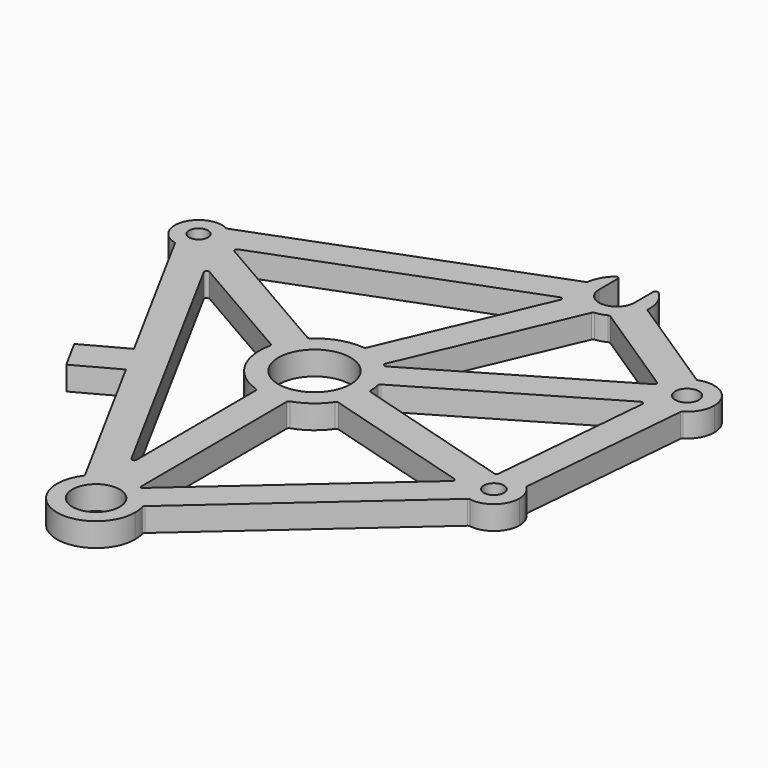
from build123d import *

# Parameters (mm, degrees)
F1_R        = 0.8
F1_R_2      = 1.5
F1_R_3      = 1
F1_R_4      = 0.85
F1_R_5      = 2
F1_R_6      = 3.05
F2_DEPTH    = 2
F4_DEPTH    = 2.001
F5_T1_DEPTH = 2
F5_T3_DEPTH = 4.0603808135


# Not quite as in the source:
# - a fillet or chamfer that OpenCascade refuses, or shapes differently, is made with other operations: its cross-section is extruded or revolved along the edge and cut away or added


with BuildPart() as f2:
    # F1 (on Top) → F2 (new body)
    with BuildSketch(Plane.XY):
        with BuildLine():
            ThreePointArc((5.1588517672, 41.7551647468), (5.8189357702, 41.1743283067), (6.1661273036, 40.3665288884))
            Line((6.1661273036, 40.3665288884), (7.2214972283, 39.7576616241))
            Line((7.2214972283, 39.7576616241), (28.9007343827, 47.9973716865))
            Line((28.9007343827, 47.9973716865), (29.1292494513, 48.531429375))
            ThreePointArc((29.1292494513, 48.531429375), (28.6106135221, 49.5207693713), (28.5200074656, 50.6341279828))
            Line((28.5200074656, 50.6341279828), (5.1588517672, 41.7551647468))
        make_face()
        with BuildLine():
            Line((42.9265921342, 44.2277120811), (34.0866325696, 50.0267255555))
            ThreePointArc((34.0866325696, 50.0267255555), (33.6412025938, 48.7641710985), (32.6605057325, 47.8527517184))
            Line((32.6605057325, 47.8527517184), (41.3390492003, 42.1596272035))
            Line((41.3390492003, 42.1596272035), (41.5054041139, 42.257574489))
            ThreePointArc((41.5054041139, 42.257574489), (41.9346789885, 43.4455770228), (42.9265921342, 44.2277120811))
        make_face()
        with BuildLine():
            Line((43.6434620305, 25.2933980565), (44.9307446243, 40.097147885))
            ThreePointArc((44.9307446243, 40.097147885), (43.8873688977, 39.8016600174), (42.8245714122, 40.0170839983))
            Line((42.8245714122, 40.0170839983), (42.2864184602, 39.7002275873))
            Line((42.2864184602, 39.7002275873), (41.0532365012, 25.518635059))
            ThreePointArc((41.0532365012, 25.518635059), (42.3862536752, 25.8419172646), (43.6434620305, 25.2933980565))
        make_face()
        with BuildLine():
            Line((39.5736067493, 23.1147203388), (23.9127614663, 9.2822986167))
            ThreePointArc((23.9127614663, 9.2822986167), (24.9733654225, 8.4845968706), (25.6339590007, 7.3335864657))
            Line((25.6339590007, 7.3335864657), (41.7771062071, 21.5920007495))
            ThreePointArc((41.7771062071, 21.5920007495), (40.8113081392, 22.0586484485), (40.1911511893, 22.9338234826))
            Line((40.1911511893, 22.9338234826), (39.5736067493, 23.1147203388))
        make_face()
        with BuildLine():
            ThreePointArc((6.0825746745, 39.3247870004), (6.1704249985, 39.6573262113), (6.2, 40))
            ThreePointArc((6.2, 40), (6.1915138221, 40.184045365), (6.1661273036, 40.3665288884))
            ThreePointArc((6.1661273036, 40.3665288884), (5.8189357702, 41.1743283067), (5.1588517672, 41.7551647468))
            ThreePointArc((5.1588517672, 41.7551647468), (2.3247456616, 40.6952849534), (3.782863546, 38.0439843613))
            ThreePointArc((3.782863546, 38.0439843613), (4.3297316575, 38.004212011), (4.8668489245, 38.1144463646))
            ThreePointArc((4.8668489245, 38.1144463646), (5.5958497172, 38.5676580133), (6.0677200026, 39.2847224372))
            ThreePointArc((6.0677200026, 39.2847224372), (6.0752543384, 39.3047150466), (6.0825746745, 39.3247870004))
        make_face()
        with Locations((4.2, 40)):
            Circle(F1_R, mode=Mode.SUBTRACT)
        with BuildLine():
            ThreePointArc((34.1, 50.3), (31.4673632334, 53.094993658), (28.5200074656, 50.6341279828))
            ThreePointArc((28.5200074656, 50.6341279828), (28.6106135221, 49.5207693713), (29.1292494513, 48.531429375))
            ThreePointArc((29.1292494513, 48.531429375), (29.2798350863, 48.3612030221), (29.443730373, 48.2037502363))
            ThreePointArc((29.443730373, 48.2037502363), (30.4109250017, 47.6449019515), (31.5196205494, 47.5086263571))
            ThreePointArc((31.5196205494, 47.5086263571), (32.1085822981, 47.6192921332), (32.6605057325, 47.8527517184))
            ThreePointArc((32.6605057325, 47.8527517184), (33.6412025938, 48.7641710985), (34.0866325696, 50.0267255555))
            ThreePointArc((34.0866325696, 50.0267255555), (34.0966561457, 50.1631994059), (34.1, 50.3))
        make_face()
        with Locations((31.3, 50.3)):
            Circle(F1_R_2, mode=Mode.SUBTRACT)
        with BuildLine():
            ThreePointArc((46.1, 42.1), (45.080851652, 44.0103452687), (42.9265921342, 44.2277120811))
            ThreePointArc((42.9265921342, 44.2277120811), (41.9346789885, 43.4455770228), (41.5054041139, 42.257574489))
            ThreePointArc((41.5054041139, 42.257574489), (41.5006748227, 42.155711122), (41.5004652971, 42.053738244))
            ThreePointArc((41.5004652971, 42.053738244), (41.730713723, 41.0959809246), (42.340519095, 40.3223848876))
            ThreePointArc((42.340519095, 40.3223848876), (42.5730125438, 40.1546204015), (42.8245714122, 40.0170839983))
            ThreePointArc((42.8245714122, 40.0170839983), (43.8873688977, 39.8016600174), (44.9307446243, 40.097147885))
            ThreePointArc((44.9307446243, 40.097147885), (45.7862921029, 40.9404122793), (46.1, 42.1))
        make_face()
        with Locations((43.8, 42.1)):
            Circle(F1_R_3, mode=Mode.SUBTRACT)
        with BuildLine():
            ThreePointArc((40.1911511893, 22.9338234826), (40.8113081392, 22.0586484485), (41.7771062071, 21.5920007495))
            ThreePointArc((41.7771062071, 21.5920007495), (43.5625854735, 22.0369122611), (44.35, 23.7))
            ThreePointArc((44.35, 23.7), (44.1654443983, 24.5715092181), (43.6434620305, 25.2933980565))
            ThreePointArc((43.6434620305, 25.2933980565), (42.3862536752, 25.8419172646), (41.0532365012, 25.518635059))
            ThreePointArc((41.0532365012, 25.518635059), (40.9868167512, 25.475017297), (40.9220541458, 25.4289749546))
            ThreePointArc((40.9220541458, 25.4289749546), (40.2457819942, 24.5963994566), (40.0559086727, 23.5407129006))
            ThreePointArc((40.0559086727, 23.5407129006), (40.1014751279, 23.2323533801), (40.1911511893, 22.9338234826))
        make_face()
        with Locations((42.2, 23.7)):
            Circle(F1_R_4, mode=Mode.SUBTRACT)
        with BuildLine():
            ThreePointArc((22.1949878763, 9.5858739483), (21.6807151801, 9.4966814642), (21.1869382745, 9.3275186052))
            ThreePointArc((21.1869382745, 9.3275186052), (20.4876667271, 8.9154377834), (19.9101314198, 8.3451358725))
            ThreePointArc((19.9101314198, 8.3451358725), (21.4175412975, 3.1825838973), (25.8, 6.3))
            ThreePointArc((25.8, 6.3), (25.7582253377, 6.8234191904), (25.6339590007, 7.3335864657))
            ThreePointArc((25.6339590007, 7.3335864657), (24.9733654225, 8.4845968706), (23.9127614663, 9.2822986167))
            ThreePointArc((23.9127614663, 9.2822986167), (23.8501326105, 9.3111695293), (23.786914122, 9.3387253977))
            ThreePointArc((23.786914122, 9.3387253977), (23.0062642444, 9.5609349142), (22.1949878763, 9.5858739483))
        make_face()
        with Locations((22.5, 6.3)):
            Circle(F1_R_5, mode=Mode.SUBTRACT)
        with BuildLine():
            Line((7.2214972283, 39.7576616241), (6.0825746745, 39.3247870004))
            ThreePointArc((6.0825746745, 39.3247870004), (6.0752543384, 39.3047150466), (6.0677200026, 39.2847224372))
            Line((6.0677200026, 39.2847224372), (7.5409732288, 36.5716823429))
            Line((7.5409732288, 36.5716823429), (17.8832035005, 30.6050110324))
            ThreePointArc((17.8832035005, 30.6050110324), (18.3722370249, 31.8237094087), (19.1824818795, 32.8570935561))
            Line((19.1824818795, 32.8570935561), (7.2214972283, 39.7576616241))
        make_face()
        with BuildLine():
            ThreePointArc((6.1661273036, 40.3665288884), (6.1915138221, 40.184045365), (6.2, 40))
            ThreePointArc((6.2, 40), (6.1704249985, 39.6573262113), (6.0825746745, 39.3247870004))
            Line((6.0825746745, 39.3247870004), (7.2214972283, 39.7576616241))
            Line((7.2214972283, 39.7576616241), (6.1661273036, 40.3665288884))
        make_face()
        with BuildLine():
            Line((7.5409732288, 36.5716823429), (6.0677200026, 39.2847224372))
            ThreePointArc((6.0677200026, 39.2847224372), (5.5958497172, 38.5676580133), (4.8668489245, 38.1144463646))
            Line((4.8668489245, 38.1144463646), (7.5409732288, 36.5716823429))
        make_face()
        with BuildLine():
            ThreePointArc((4.8668489245, 38.1144463646), (4.3297316575, 38.004212011), (3.782863546, 38.0439843613))
            Line((3.782863546, 38.0439843613), (11.1306870545, 24.5127465342))
            Line((11.1306870545, 24.5127465342), (12.5623079112, 21.8763736997))
            Line((12.5623079112, 21.8763736997), (19.9101314198, 8.3451358725))
            ThreePointArc((19.9101314198, 8.3451358725), (20.4876667271, 8.9154377834), (21.1869382745, 9.3275186052))
            Line((21.1869382745, 9.3275186052), (21.1777502182, 11.4591476685))
            Line((21.1777502182, 11.4591476685), (7.5409732288, 36.5716823429))
            Line((7.5409732288, 36.5716823429), (4.8668489245, 38.1144463646))
        make_face()
        with BuildLine():
            Line((22.1949878763, 9.5858739483), (21.1777502182, 11.4591476685))
            Line((21.1777502182, 11.4591476685), (21.1869382745, 9.3275186052))
            ThreePointArc((21.1869382745, 9.3275186052), (21.6807151801, 9.4966814642), (22.1949878763, 9.5858739483))
        make_face()
        with BuildLine():
            Line((21.119255789, 25.0298552298), (21.1777502182, 11.4591476685))
            Line((21.1777502182, 11.4591476685), (22.1949878763, 9.5858739483))
            ThreePointArc((22.1949878763, 9.5858739483), (23.0062642444, 9.5609349142), (23.786914122, 9.3387253977))
            Line((23.786914122, 9.3387253977), (23.7192316366, 25.0410620223))
            ThreePointArc((23.7192316366, 25.0410620223), (22.4200429173, 24.8500431957), (21.119255789, 25.0298552298))
        make_face()
        with BuildLine():
            Line((40.0559086727, 23.5407129006), (39.5736067493, 23.1147203388))
            Line((39.5736067493, 23.1147203388), (40.1911511893, 22.9338234826))
            ThreePointArc((40.1911511893, 22.9338234826), (40.1014751279, 23.2323533801), (40.0559086727, 23.5407129006))
        make_face()
        with BuildLine():
            ThreePointArc((27.0499939641, 29.4925077351), (26.8624824403, 28.192808174), (26.3190910076, 26.9973562631))
            Line((26.3190910076, 26.9973562631), (39.5736067493, 23.1147203388))
            Line((39.5736067493, 23.1147203388), (40.0559086727, 23.5407129006))
            ThreePointArc((40.0559086727, 23.5407129006), (40.2457819942, 24.5963994566), (40.9220541458, 25.4289749546))
            Line((40.9220541458, 25.4289749546), (27.0499939641, 29.4925077351))
        make_face()
        with BuildLine():
            Line((29.1292494513, 48.531429375), (28.9007343827, 47.9973716865))
            Line((28.9007343827, 47.9973716865), (29.443730373, 48.2037502363))
            ThreePointArc((29.443730373, 48.2037502363), (29.2798350863, 48.3612030221), (29.1292494513, 48.531429375))
        make_face()
        with BuildLine():
            Line((29.443730373, 48.2037502363), (28.9007343827, 47.9973716865))
            Line((28.9007343827, 47.9973716865), (22.9611178394, 34.116020664))
            ThreePointArc((22.9611178394, 34.116020664), (24.229243859, 33.7750867716), (25.3514889375, 33.0932176461))
            Line((25.3514889375, 33.0932176461), (31.5196205494, 47.5086263571))
            ThreePointArc((31.5196205494, 47.5086263571), (30.4109250017, 47.6449019515), (29.443730373, 48.2037502363))
        make_face()
        with BuildLine():
            ThreePointArc((22.9611178394, 34.116020664), (20.9301904957, 33.9115938187), (19.1824818795, 32.8570935561))
            ThreePointArc((19.1824818795, 32.8570935561), (18.3722370249, 31.8237094087), (17.8832035005, 30.6050110324))
            ThreePointArc((17.8832035005, 30.6050110324), (18.378375934, 27.1656821399), (21.119255789, 25.0298552298))
            ThreePointArc((21.119255789, 25.0298552298), (22.4200429173, 24.8500431957), (23.7192316366, 25.0410620223))
            ThreePointArc((23.7192316366, 25.0410620223), (25.1958501069, 25.7843947761), (26.3190910076, 26.9973562631))
            ThreePointArc((26.3190910076, 26.9973562631), (26.8624824403, 28.192808174), (27.0499939641, 29.4925077351))
            ThreePointArc((27.0499939641, 29.4925077351), (27.049998491, 29.4962538663), (27.05, 29.5))
            ThreePointArc((27.05, 29.5), (27.0140701204, 30.0769375391), (26.9068357316, 30.6449592518))
            ThreePointArc((26.9068357316, 30.6449592518), (26.40703107, 31.8592799758), (25.5876684333, 32.8854497425))
            ThreePointArc((25.5876684333, 32.8854497425), (25.471336058, 32.991331382), (25.3514889375, 33.0932176461))
            ThreePointArc((25.3514889375, 33.0932176461), (24.229243859, 33.7750867716), (22.9611178394, 34.116020664))
        make_face()
        with Locations((22.4, 29.5)):
            Circle(F1_R_6, mode=Mode.SUBTRACT)
        with BuildLine():
            Line((41.5054041139, 42.257574489), (41.3390492003, 42.1596272035))
            Line((41.3390492003, 42.1596272035), (41.5004652971, 42.053738244))
            ThreePointArc((41.5004652971, 42.053738244), (41.5006748227, 42.155711122), (41.5054041139, 42.257574489))
        make_face()
        with BuildLine():
            Line((42.340519095, 40.3223848876), (42.2864184602, 39.7002275873))
            Line((42.2864184602, 39.7002275873), (42.8245714122, 40.0170839983))
            ThreePointArc((42.8245714122, 40.0170839983), (42.5730125438, 40.1546204015), (42.340519095, 40.3223848876))
        make_face()
        with BuildLine():
            Line((41.3390492003, 42.1596272035), (25.5876684333, 32.8854497425))
            ThreePointArc((25.5876684333, 32.8854497425), (26.40703107, 31.8592799758), (26.9068357316, 30.6449592518))
            Line((26.9068357316, 30.6449592518), (42.2864184602, 39.7002275873))
            Line((42.2864184602, 39.7002275873), (42.340519095, 40.3223848876))
            ThreePointArc((42.340519095, 40.3223848876), (41.730713723, 41.0959809246), (41.5004652971, 42.053738244))
            Line((41.5004652971, 42.053738244), (41.3390492003, 42.1596272035))
        make_face()
        Polygon((12.5623079112, 21.8763736997), (11.1306870545, 24.5127465342), (7.6155232752, 22.6039187252), (9.0471441319, 19.9675458907), align=None)
    extrude(amount=-F2_DEPTH)

    # F3 (on face) → F4 (cut, through all)
    with BuildSketch(Plane.XY):
        with BuildLine():
            Line((29.8, 52.6643180835), (29.8, 50.3))
            ThreePointArc((29.8, 50.3), (31.3, 51.8), (32.8, 50.3))
            Line((32.8, 50.3), (32.8, 52.6643180835))
            ThreePointArc((32.8, 52.6643180835), (31.3, 53.1), (29.8, 52.6643180835))
        make_face()
    extrude(amount=-F4_DEPTH, mode=Mode.SUBTRACT)

    # F5: fillet of radius 0.2 on 35 edges, made by hand

    # F5_s2 → F5_t1 (join)
    with BuildSketch(Plane.XY.offset(-2)):
        with BuildLine():
            ThreePointArc((7.6152873474, 39.9073309314), (7.4869831486, 39.736368397), (7.586398465, 39.5471416799))
            Line((7.586398465, 39.5471416799), (7.2214972283, 39.7576616241))
            Line((7.2214972283, 39.7576616241), (7.6152873474, 39.9073309314))
        make_face()
        with BuildLine():
            ThreePointArc((8.1549136009, 36.2174859744), (7.9153841385, 36.1874830559), (7.8792109212, 35.9488074668))
            Line((7.8792109212, 35.9488074668), (7.5409732288, 36.5716823429))
            Line((7.5409732288, 36.5716823429), (8.1549136009, 36.2174859744))
        make_face()
        with BuildLine():
            ThreePointArc((20.7985689859, 12.157421304), (21.0239808003, 12.0591244239), (21.174325317, 12.2537247554))
            Line((21.174325317, 12.2537247554), (21.1777502182, 11.4591476685))
            Line((21.1777502182, 11.4591476685), (20.7985689859, 12.157421304))
        make_face()
        with BuildLine():
            ThreePointArc((19.8343096871, 8.2452750848), (19.8723110487, 8.349886538), (19.8485108874, 8.4586119349))
            Line((19.8485108874, 8.4586119349), (19.9101314198, 8.3451358725))
            ThreePointArc((19.9101314198, 8.3451358725), (19.8717462329, 8.295565618), (19.8343096871, 8.2452750848))
        make_face()
        with BuildLine():
            ThreePointArc((25.7307406523, 7.4190687367), (25.6711167797, 7.3250865393), (25.6709610076, 7.2137867848))
            ThreePointArc((25.6709610076, 7.2137867848), (25.6530290307, 7.273862378), (25.6339590007, 7.3335864657))
            Line((25.6339590007, 7.3335864657), (25.7307406523, 7.4190687367))
        make_face()
        with BuildLine():
            ThreePointArc((20.9809292738, 25.0718244983), (21.0812054105, 24.9995965527), (21.1198921159, 24.8822273979))
            Line((21.1198921159, 24.8822273979), (21.119255789, 25.0298552298))
            ThreePointArc((21.119255789, 25.0298552298), (21.0499294357, 25.0503023168), (20.9809292738, 25.0718244983))
        make_face()
        with BuildLine():
            ThreePointArc((17.7553292124, 30.6787846601), (17.8380565482, 30.5869785186), (17.85103896, 30.4640816648))
            ThreePointArc((17.85103896, 30.4640816648), (17.8665735681, 30.5346713424), (17.8832035005, 30.6050110324))
            Line((17.8832035005, 30.6050110324), (17.7553292124, 30.6787846601))
        make_face()
        with BuildLine():
            ThreePointArc((3.6998231735, 38.0635539919), (3.77290973, 38.0275334575), (3.8255636798, 37.9653507815))
            Line((3.8255636798, 37.9653507815), (3.782863546, 38.0439843613))
            ThreePointArc((3.782863546, 38.0439843613), (3.7412389988, 38.0533263387), (3.6998231735, 38.0635539919))
        make_face()
        with BuildLine():
            ThreePointArc((5.2424934778, 41.7869547697), (5.1620285352, 41.7741283656), (5.0831253359, 41.7944608218))
            ThreePointArc((5.0831253359, 41.7944608218), (5.1211981098, 41.7752166185), (5.1588517672, 41.7551647468))
            Line((5.1588517672, 41.7551647468), (5.2424934778, 41.7869547697))
        make_face()
        with BuildLine():
            ThreePointArc((28.4095590818, 50.5921494458), (28.4935155026, 50.6527240866), (28.5359365753, 50.7471614748))
            ThreePointArc((28.5359365753, 50.7471614748), (28.5273959421, 50.6907259119), (28.5200074656, 50.6341279828))
            Line((28.5200074656, 50.6341279828), (28.4095590818, 50.5921494458))
        make_face()
        with BuildLine():
            ThreePointArc((28.4605609872, 47.8300733111), (28.6759140893, 47.7816066752), (28.7154912953, 47.5644440215))
            Line((28.7154912953, 47.5644440215), (28.9007343827, 47.9973716865))
            Line((28.9007343827, 47.9973716865), (28.4605609872, 47.8300733111))
        make_face()
        with BuildLine():
            ThreePointArc((34.0954553724, 50.1405344523), (34.1165116032, 50.0391707367), (34.1854286918, 49.9619152993))
            Line((34.1854286918, 49.9619152993), (34.0866325696, 50.0267255555))
            ThreePointArc((34.0866325696, 50.0267255555), (34.0916240012, 50.0835850382), (34.0954553724, 50.1405344523))
        make_face()
        with BuildLine():
            ThreePointArc((42.8407758516, 44.2840075625), (42.9271443802, 44.2526021174), (43.0184396827, 44.2631374137))
            ThreePointArc((43.0184396827, 44.2631374137), (42.9723263564, 44.2459162005), (42.9265921342, 44.2277120811))
            Line((42.9265921342, 44.2277120811), (42.8407758516, 44.2840075625))
        make_face()
        with BuildLine():
            ThreePointArc((45.0154135176, 40.1473684471), (44.9506371038, 40.082177643), (44.9218535319, 39.9949003223))
            Line((44.9218535319, 39.9949003223), (44.9307446243, 40.097147885))
            ThreePointArc((44.9307446243, 40.097147885), (44.9733477886, 40.1218051241), (45.0154135176, 40.1473684471))
        make_face()
        with BuildLine():
            ThreePointArc((41.9520853542, 39.5033772539), (42.1602543232, 39.5001952749), (42.2528078794, 39.3137059082))
            Line((42.2528078794, 39.3137059082), (42.2864184602, 39.7002275873))
            Line((42.2864184602, 39.7002275873), (41.9520853542, 39.5033772539))
        make_face()
        with BuildLine():
            ThreePointArc((41.0701434494, 42.3360293761), (41.1603827047, 42.163956174), (41.0619157925, 41.996455197))
            Line((41.0619157925, 41.996455197), (41.3390492003, 42.1596272035))
            Line((41.3390492003, 42.1596272035), (41.0701434494, 42.3360293761))
        make_face()
        with BuildLine():
            ThreePointArc((43.6518261956, 25.3895859545), (43.6633730003, 25.3032077532), (43.7105573504, 25.2299400286))
            ThreePointArc((43.7105573504, 25.2299400286), (43.6773504513, 25.2620293352), (43.6434620305, 25.2933980565))
            Line((43.6434620305, 25.2933980565), (43.6518261956, 25.3895859545))
        make_face()
        with BuildLine():
            ThreePointArc((41.8680223308, 21.5757846561), (41.7810575454, 21.5701589596), (41.7047408769, 21.5280841635))
            Line((41.7047408769, 21.5280841635), (41.7771062071, 21.5920007495))
            ThreePointArc((41.7771062071, 21.5920007495), (41.8224771908, 21.5834044958), (41.8680223308, 21.5757846561))
        make_face()
        with BuildLine():
            ThreePointArc((39.2257695535, 23.2166120426), (39.3647578651, 23.0681793251), (39.3019460595, 22.8747763793))
            Line((39.3019460595, 22.8747763793), (39.5736067493, 23.1147203388))
            Line((39.5736067493, 23.1147203388), (39.2257695535, 23.2166120426))
        make_face()
        with BuildLine():
            ThreePointArc((23.0191930682, 34.2517470413), (22.9378544501, 34.1587082918), (22.8173670954, 34.1312314461))
            ThreePointArc((22.8173670954, 34.1312314461), (22.8893015776, 34.1241846812), (22.9611178394, 34.116020664))
            Line((22.9611178394, 34.116020664), (23.0191930682, 34.2517470413))
        make_face()
        with BuildLine():
            ThreePointArc((19.0546075915, 32.9308671838), (19.1754941828, 32.905203752), (19.288384986, 32.9554814433))
            ThreePointArc((19.288384986, 32.9554814433), (19.2350510901, 32.9066990471), (19.1824818795, 32.8570935561))
            Line((19.1824818795, 32.8570935561), (19.0546075915, 32.9308671838))
        make_face()
        with BuildLine():
            ThreePointArc((23.8571912146, 25.084222179), (23.7575414471, 25.0111324839), (23.7198679635, 24.8934341903))
            Line((23.7198679635, 24.8934341903), (23.7192316366, 25.0410620223))
            ThreePointArc((23.7192316366, 25.0410620223), (23.7883791492, 25.0621059794), (23.8571912146, 25.084222179))
        make_face()
        with BuildLine():
            ThreePointArc((26.2394077419, 26.8767485459), (26.3372386428, 26.9522554628), (26.4607668631, 26.9558552549))
            Line((26.4607668631, 26.9558552549), (26.3190910076, 26.9973562631))
            ThreePointArc((26.3190910076, 26.9973562631), (26.2797180654, 26.9367427493), (26.2394077419, 26.8767485459))
        make_face()
        with BuildLine():
            ThreePointArc((23.7863575432, 9.4678516807), (23.8177871956, 9.3610816635), (23.9014210748, 9.287644385))
            ThreePointArc((23.9014210748, 9.287644385), (23.8444102239, 9.3137287784), (23.786914122, 9.3387253977))
            Line((23.786914122, 9.3387253977), (23.7863575432, 9.4678516807))
        make_face()
        with BuildLine():
            ThreePointArc((23.7984494043, 9.3338142897), (23.9089161507, 9.3202217342), (24.0095431179, 9.3677808877))
            Line((24.0095431179, 9.3677808877), (23.9127614663, 9.2822986167))
            ThreePointArc((23.9127614663, 9.2822986167), (23.8558501253, 9.3085994146), (23.7984494043, 9.3338142897))
        make_face()
        with BuildLine():
            ThreePointArc((27.0479800053, 29.6370469625), (27.0896079095, 29.5206884764), (27.1916698195, 29.4510067269))
            Line((27.1916698195, 29.4510067269), (27.0499939641, 29.4925077351))
            ThreePointArc((27.0499939641, 29.4925077351), (27.049548675, 29.5647851752), (27.0479800053, 29.6370469625))
        make_face()
        with BuildLine():
            ThreePointArc((26.9402467942, 30.5043201917), (26.9521405733, 30.6273271741), (27.0340518186, 30.7198621815))
            Line((27.0340518186, 30.7198621815), (26.9068357316, 30.6449592518))
            ThreePointArc((26.9068357316, 30.6449592518), (26.9240877968, 30.5747695596), (26.9402467942, 30.5043201917))
        make_face()
        with BuildLine():
            ThreePointArc((40.8293968182, 25.4561170001), (40.9163574726, 25.4504278048), (40.9974822397, 25.4822600922))
            ThreePointArc((40.9974822397, 25.4822600922), (40.9594820589, 25.4560225619), (40.9220541458, 25.4289749546))
            Line((40.9220541458, 25.4289749546), (40.8293968182, 25.4561170001))
        make_face()
        with BuildLine():
            ThreePointArc((40.9761948849, 25.4677106778), (41.0353176138, 25.5317343085), (41.0616006663, 25.6148229571))
            Line((41.0616006663, 25.6148229571), (41.0532365012, 25.518635059))
            ThreePointArc((41.0532365012, 25.518635059), (41.0144422362, 25.4935865713), (40.9761948849, 25.4677106778))
        make_face()
        with BuildLine():
            ThreePointArc((31.6332130872, 47.5198976568), (31.5371124385, 47.4813926831), (31.4731393222, 47.3999960733))
            Line((31.4731393222, 47.3999960733), (31.5196205494, 47.5086263571))
            ThreePointArc((31.5196205494, 47.5086263571), (31.5764742628, 47.5136830794), (31.6332130872, 47.5198976568))
        make_face()
        with BuildLine():
            ThreePointArc((32.5596264709, 47.7993318585), (32.6609901865, 47.8203880893), (32.7593018546, 47.7879414622))
            Line((32.7593018546, 47.7879414622), (32.6605057325, 47.8527517184))
            ThreePointArc((32.6605057325, 47.8527517184), (32.6103383575, 47.8255276544), (32.5596264709, 47.7993318585))
        make_face()
        with BuildLine():
            ThreePointArc((25.4095641662, 33.2289440234), (25.3984297346, 33.1058659826), (25.4617506654, 32.9997403993))
            ThreePointArc((25.4617506654, 32.9997403993), (25.406983061, 33.046907508), (25.3514889375, 33.0932176461))
            Line((25.3514889375, 33.0932176461), (25.4095641662, 33.2289440234))
        make_face()
        with BuildLine():
            ThreePointArc((25.4808983556, 32.9828961114), (25.5942298904, 32.9336199214), (25.7148845204, 32.9603526723))
            Line((25.7148845204, 32.9603526723), (25.5876684333, 32.8854497425))
            ThreePointArc((25.5876684333, 32.8854497425), (25.5346620784, 32.9345878435), (25.4808983556, 32.9828961114))
        make_face()
    extrude(amount=F5_T1_DEPTH)

    # F5_s4 → F5_t3 (cut)
    with BuildSketch(Plane.XY.offset(-3.0301904067)):
        with BuildLine():
            ThreePointArc((29.4692307692, 52.4185570617), (29.6832050294, 52.4491021791), (29.8, 52.2672315573))
            Line((29.8, 52.2672315573), (29.8, 52.6643180835))
            ThreePointArc((29.8, 52.6643180835), (29.6300881649, 52.5475307479), (29.4692307692, 52.4185570617))
        make_face()
        with BuildLine():
            ThreePointArc((32.8, 52.2672315573), (32.9167949706, 52.4491021791), (33.1307692308, 52.4185570617))
            ThreePointArc((33.1307692308, 52.4185570617), (32.9699118351, 52.5475307479), (32.8, 52.6643180835))
            Line((32.8, 52.6643180835), (32.8, 52.2672315573))
        make_face()
    extrude(amount=F5_T3_DEPTH, mode=Mode.SUBTRACT)


solid = f2.part
